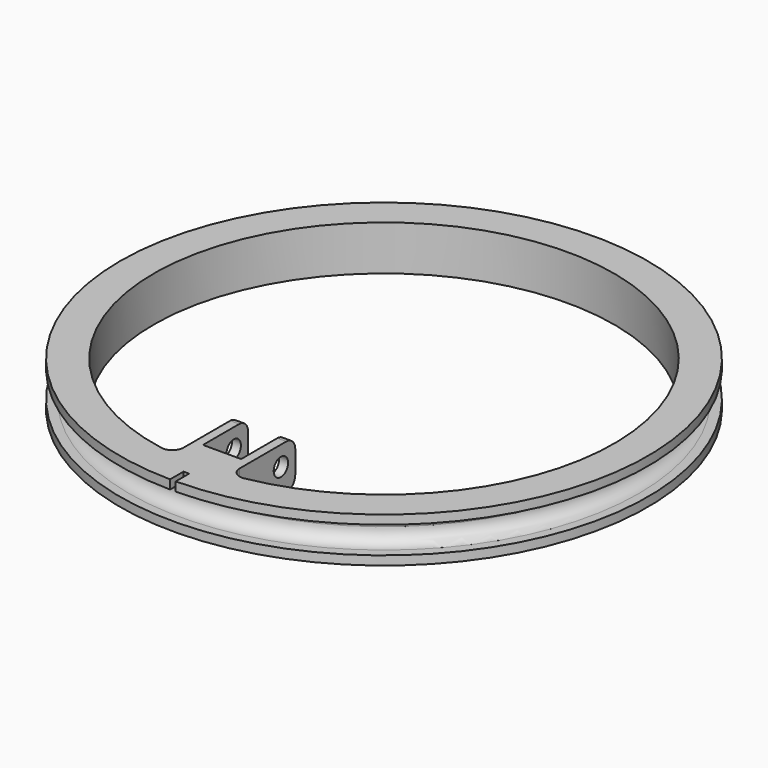
from build123d import *

# Parameters (mm, degrees)
F2_R      = 2.4
F3_R      = 2.39999
F5_W      = 10
F5_H      = 8
F7_R      = 1.6
F8_DEPTH  = 5
F7_W      = 4.6828329376
F7_H      = 1.903038422
F9_DEPTH  = 3.4
F10_R     = 2
F11_W     = 4
F11_H     = 4
F12_DEPTH = 0.5


# Not quite as in the source:
# - a fillet or chamfer is up to 0.001 mm smaller than in the source, because OpenCascade refuses the exact size
# - a feature names something its author has since deleted; it is built from what else it names


with BuildPart() as f1:
    # F0 (on Front) → F1 (revolve)
    with BuildSketch(Plane.XZ):
        Polygon((-41, 5), (-47, 5), (-47, 3.4), (-43, 3.4), (-43, -1.4), (-47, -1.4), (-47, -3), (-41, -3), align=None)
    revolve(axis=Axis((0, 0, 0.7178727537), (0, 0, 1)))

    # F2
    f2_edges = [f1.edges().sort_by_distance(p)[0] for p in [
        (43, 0, 3.4),
    ]]
    fillet(f2_edges, radius=F2_R)

    # F3 (radius 2.4 in the source; OpenCascade refuses exactly that, so slightly less here)
    f3_edges = [f1.edges().sort_by_distance(p)[0] for p in [
        (43, 0, -1.4),
    ]]
    fillet(f3_edges, radius=F3_R)

    # F5 (on offset) → F6 (join, up to the next surface of F1)
    with BuildSketch(Plane.XZ.offset(26)):
        with Locations((0, 1)):
            Rectangle(F5_W, F5_H)
    extrude(until=Until.NEXT)

    # F7 (on Right) → F8 (cut, symmetric)
    with BuildSketch(Plane.YZ):
        with Locations((-29.2, 1.5)):
            Circle(F7_R)
    extrude(amount=F8_DEPTH, both=True, mode=Mode.SUBTRACT)

    # F7 (on Right) → F9 (cut, symmetric)
    with BuildSketch(Plane.YZ):
        Polygon((-26, 5.4147794951), (-36.4011118985, 5.4147794951), (-30.6828329376, -1.4), (-26, -1.4), (-26, 3.0355471618), align=None)
        with Locations((-29.2, 1.5)):
            Circle(F7_R, mode=Mode.SUBTRACT)
        with Locations((-28.3414164688, -2.351519211)):
            Rectangle(F7_W, F7_H)
    extrude(amount=F9_DEPTH, both=True, mode=Mode.SUBTRACT)

    # F10
    f10_edges = [f1.edges().sort_by_distance(p)[0] for p in [
        (-4.2, -26, 5),
        (4.2, -26, 5),
        (-4.2, -26, -3),
        (4.2, -26, -3),
        (-5, -40.69398, 1),
        (5, -40.69398, 1),
    ]]
    fillet(f10_edges, radius=F10_R)

    # F11 (on Right) → F12 (cut, symmetric)
    with BuildSketch(Plane.YZ):
        with Locations((-46, 3)):
            Rectangle(F11_W, F11_H)
    extrude(amount=F12_DEPTH, both=True, mode=Mode.SUBTRACT)


solid = f1.part
